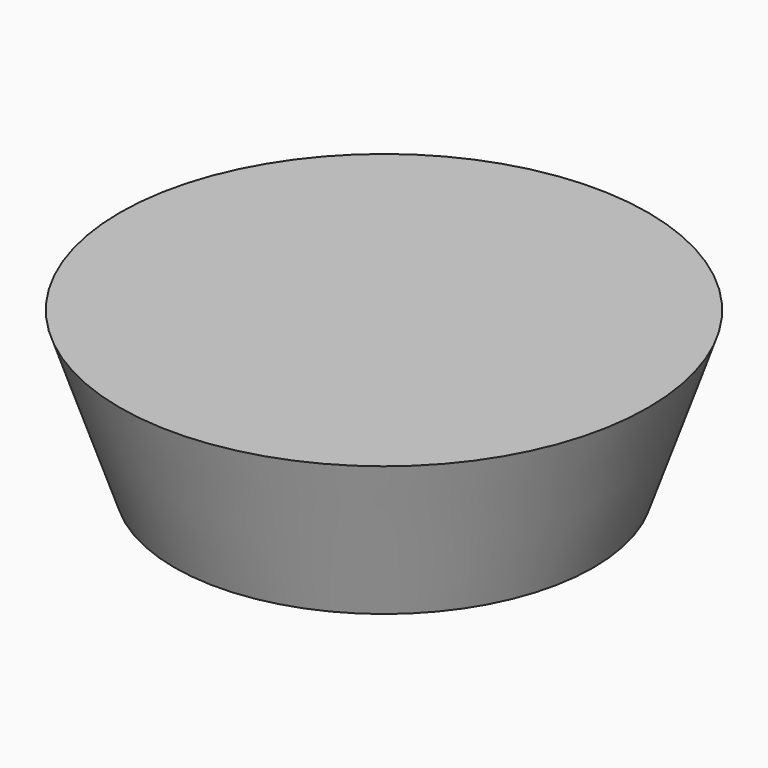
from build123d import *

# Parameters (mm, degrees)
F0_R     = 5
F1_DEPTH = 3
F2_SIZE2 = 1.032973
F2_SIZE  = 2.99999


# Not quite as in the source:
# - a fillet or chamfer is up to 0.001 mm smaller than in the source, because OpenCascade refuses the exact size


with BuildPart() as f1:
    # F0 (on Top) → F1 (new body)
    with BuildSketch(Plane.XY):
        Circle(F0_R)
    extrude(amount=F1_DEPTH)

    # F2 (size 3 and 1.0329828399 in the source; OpenCascade refuses exactly that, so slightly less here)
    f2_edges = [f1.edges().sort_by_distance(p)[0] for p in [
        (-5, 0, 0),
    ]]
    f2_side = f1.faces().sort_by_distance((-5, 0, 1.5))[0]
    chamfer(f2_edges, length=F2_SIZE, length2=F2_SIZE2, reference=f2_side)


solid = f1.part
